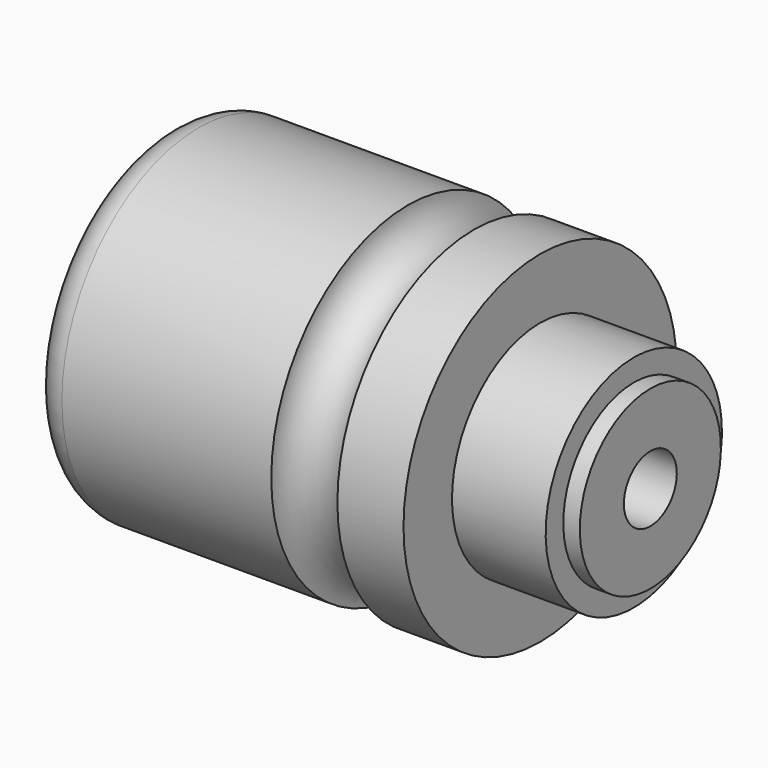
from build123d import *

# Parameters (mm, degrees)
F4_R = 5.99999


# Not quite as in the source:
# - a fillet or chamfer is up to 0.001 mm smaller than in the source, because OpenCascade refuses the exact size


with BuildPart() as f1:
    # F0 (on Front) → F1 (revolve)
    with BuildSketch(Plane.XZ):
        with BuildLine():
            Line((0, 31), (0, 0))
            Line((0, 0), (88, 0))
            Line((88, 0), (88, 16))
            Line((88, 16), (85, 16))
            Line((85, 16), (85, 20))
            Line((85, 20), (68, 20))
            Line((68, 20), (68, 31))
            Line((68, 31), (56, 31))
            ThreePointArc((56, 31), (50, 25), (44, 31))
            Line((44, 31), (0, 31))
        make_face()
    revolve(axis=Axis((56.2561290468, 0, 0), (1, 0, 0)))

    # F2 (on Front) → F3 (revolve, cut)
    with BuildSketch(Plane.XZ):
        Polygon((0, 25), (0, 0), (88, 0), (88, 6), (30, 6), (30, 16), (22, 16), (22, 20.5), (17, 20.5), (17, 12.5), (14, 12.5), (14, 16), (1.5, 16), (1.5, 25), align=None)
    revolve(axis=Axis((-8.4188580513, 0, 0), (-1, 0, 0)), mode=Mode.SUBTRACT)

    # F4 (radius 6 in the source; OpenCascade refuses exactly that, so slightly less here)
    f4_edges = [f1.edges().sort_by_distance(p)[0] for p in [
        (0, 0, -31),
    ]]
    fillet(f4_edges, radius=F4_R)


solid = f1.part
